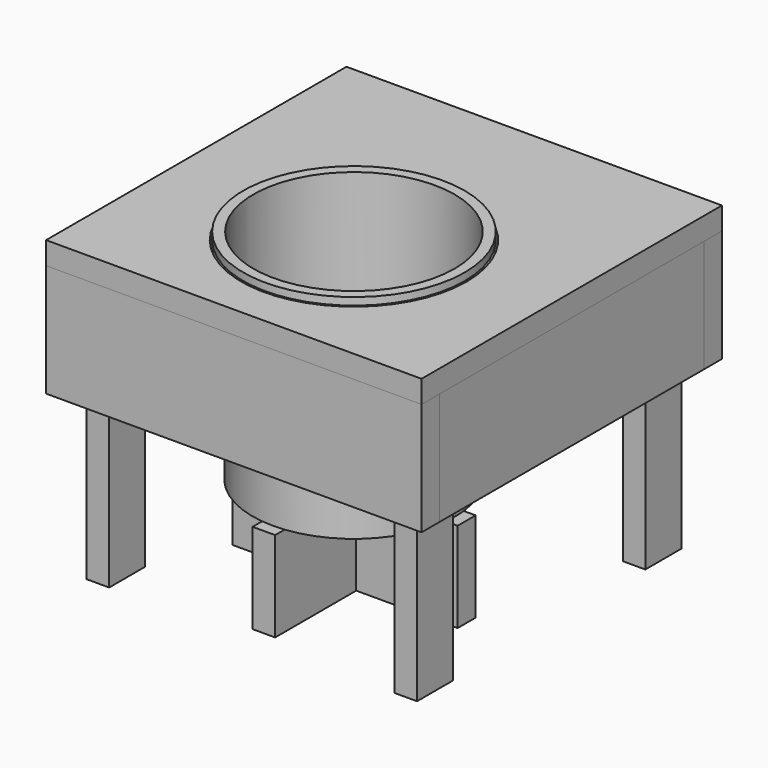
from build123d import *

# Parameters (mm, degrees)
F0_W      = 500
F0_H      = 500
F1_DEPTH  = 30
F2_W      = 30
F2_H      = 60
F19_DEPTH = 370
F20_DEPTH = 150
F3_W      = 30
F3_H      = 440
F4_DEPTH  = 150
F5_DEPTH  = 150
F6_R      = 150
F21_DEPTH = 400.001
F8_DEPTH  = 120
F7_W      = 135
F7_H      = 30
F9_DEPTH  = 120
F10_W     = 30
F10_H     = 60
F11_DEPTH = 265.001
F12_W     = 30
F12_H     = 60
F13_DEPTH = 315.001
F15_DEPTH = 280
F16_T     = -1
F17_R     = 147.5
F17_R_2   = 135
F17_R_3   = 134
F18_DEPTH = 10


with BuildPart() as f1:
    # F0 (on Top) → F1 (new body)
    with BuildSketch(Plane.XY):
        with Locations((250, 250)):
            Rectangle(F0_W, F0_H)
    extrude(amount=F1_DEPTH)

    # F6 (on face) → F21 (cut, through all)
    with BuildSketch(Plane.XY.offset(30)):
        with Locations((250, 200)):
            Circle(F6_R)
    extrude(amount=-F21_DEPTH, mode=Mode.SUBTRACT)


with BuildPart() as f19:
    # F2 (on face) → F19 (new body)
    with BuildSketch(Plane(origin=(0, 0, 0), x_dir=(1, 0, 0), z_dir=(0, 0, -1))):
        with Locations((45, -60)):
            Rectangle(F2_W, F2_H)
    extrude(amount=F19_DEPTH)


with BuildPart() as f19b:
    # F2 (on face) → F19, piece 2 (new body)
    with BuildSketch(Plane(origin=(0, 0, 0), x_dir=(1, 0, 0), z_dir=(0, 0, -1))):
        with Locations((455, -60)):
            Rectangle(F2_W, F2_H)
    extrude(amount=F19_DEPTH)


with BuildPart() as f19c:
    # F2 (on face) → F19, piece 3 (new body)
    with BuildSketch(Plane(origin=(0, 0, 0), x_dir=(1, 0, 0), z_dir=(0, 0, -1))):
        with Locations((455, -440)):
            Rectangle(F2_W, F2_H)
    extrude(amount=F19_DEPTH)


with BuildPart() as f19d:
    # F2 (on face) → F19, piece 4 (new body)
    with BuildSketch(Plane(origin=(0, 0, 0), x_dir=(1, 0, 0), z_dir=(0, 0, -1))):
        with Locations((45, -440)):
            Rectangle(F2_W, F2_H)
    extrude(amount=F19_DEPTH)


with BuildPart() as f20:
    # F3 (on face) → F20 (new body)
    with BuildSketch(Plane(origin=(0, 0, 0), x_dir=(1, 0, 0), z_dir=(0, 0, -1))):
        Polygon((0, 0), (0, -30), (30, -30), (470, -30), (500, -30), (500, 0), align=None)
    extrude(amount=F20_DEPTH)


with BuildPart() as f4:
    # F3 (on face) → F4 (new body)
    with BuildSketch(Plane(origin=(0, 0, 0), x_dir=(1, 0, 0), z_dir=(0, 0, -1))):
        with Locations((15, -250)):
            Rectangle(F3_W, F3_H)
    extrude(amount=F4_DEPTH)


with BuildPart() as f4b:
    # F3 (on face) → F4, piece 2 (new body)
    with BuildSketch(Plane(origin=(0, 0, 0), x_dir=(1, 0, 0), z_dir=(0, 0, -1))):
        with Locations((485, -250)):
            Rectangle(F3_W, F3_H)
    extrude(amount=F4_DEPTH)


with BuildPart() as f5:
    # F3 (on face) → F5 (new body)
    with BuildSketch(Plane(origin=(0, 0, 0), x_dir=(1, 0, 0), z_dir=(0, 0, -1))):
        Polygon((30, -470), (0, -470), (0, -500), (500, -500), (500, -470), (470, -470), align=None)
    extrude(amount=F5_DEPTH)


with BuildPart() as f8:
    # F7 (on face) → F8 (new body)
    with BuildSketch(Plane(origin=(0, 0, -370), x_dir=(1, 0, 0), z_dir=(0, 0, -1))):
        Polygon((250, -185), (265, -185), (265, -50), (235, -50), (235, -185), align=None)
        Polygon((235, -185), (235, -215), (250, -215), (250, -200), (250, -185), align=None)
        Polygon((250, -215), (265, -215), (265, -185), (250, -185), (250, -200), align=None)
        Polygon((235, -350), (265, -350), (265, -215), (250, -215), (235, -215), align=None)
    extrude(amount=-F8_DEPTH)

    # F10 (on face) → F11 (cut, through all)
    with BuildSketch(Plane.YZ.offset(265)):
        with Locations((200, -280)):
            Rectangle(F10_W, F10_H)
    extrude(amount=-F11_DEPTH, mode=Mode.SUBTRACT)


with BuildPart() as f9:
    # F7 (on face) → F9 (new body)
    with BuildSketch(Plane(origin=(0, 0, -370), x_dir=(1, 0, 0), z_dir=(0, 0, -1))):
        with Locations((167.5, -200)):
            Rectangle(F7_W, F7_H)
        Polygon((250, -215), (265, -215), (265, -185), (250, -185), (250, -200), align=None)
        Polygon((235, -185), (235, -215), (250, -215), (250, -200), (250, -185), align=None)
        with Locations((332.5, -200)):
            Rectangle(F7_W, F7_H)
    extrude(amount=-F9_DEPTH)

    # F12 (on face) → F13 (cut, through all)
    with BuildSketch(Plane.XZ.offset(-185)):
        with Locations((250, -340)):
            Rectangle(F12_W, F12_H)
    extrude(amount=-F13_DEPTH, mode=Mode.SUBTRACT)


with BuildPart() as f15:
    # F14 (on face) → F15 (new body)
    with BuildSketch(Plane.XY.offset(-250)):
        with BuildLine():
            Line((115.83592135, 215), (384.16407865, 215))
            ThreePointArc((384.16407865, 215), (250, 335), (115.83592135, 215))
        make_face()
        with BuildLine():
            ThreePointArc((115.83592135, 185), (250, 65), (384.16407865, 185))
            Line((384.16407865, 185), (115.83592135, 185))
        make_face()
        with BuildLine():
            ThreePointArc((384.16407865, 185), (384.7908576606, 192.488362953), (385, 200))
            ThreePointArc((385, 200), (384.7908576606, 207.511637047), (384.16407865, 215))
            Line((384.16407865, 215), (115.83592135, 215))
            ThreePointArc((115.83592135, 215), (115, 200), (115.83592135, 185))
            Line((115.83592135, 185), (384.16407865, 185))
        make_face()
    extrude(amount=F15_DEPTH)

    # F16
    f16_openings = [f15.faces().sort_by_distance(p)[0] for p in [
        (250, 200, 30),
    ]]
    offset(amount=F16_T, openings=f16_openings)

    # F17 (on face) → F18 (join)
    with BuildSketch(Plane.XY.offset(30)):
        with Locations((250, 200)):
            Circle(F17_R)
        with Locations((250, 200)):
            Circle(F17_R_2, mode=Mode.SUBTRACT)
        with Locations((250, 200)):
            Circle(F17_R_2)
        with Locations((250, 200)):
            Circle(F17_R_3, mode=Mode.SUBTRACT)
    extrude(amount=F18_DEPTH)


solid = Compound([f1.part, f19.part, f19b.part, f19c.part, f19d.part, f20.part, f4.part, f4b.part, f5.part, f8.part, f9.part, f15.part])
